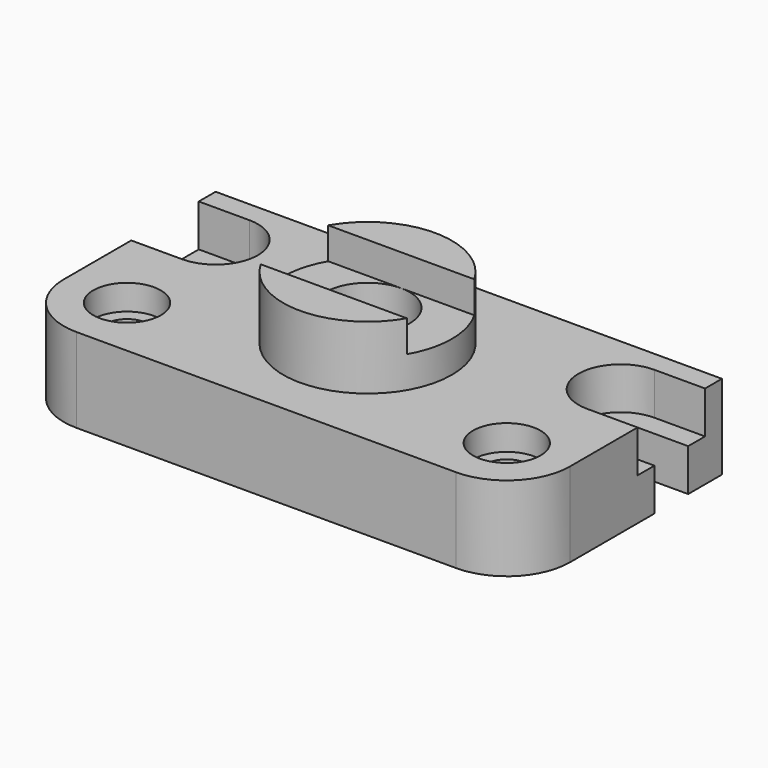
from build123d import *

# Parameters (mm, degrees)
F1_DEPTH        = 20
F2_R            = 20
F3_DEPTH        = 15
F6_DEPTH        = 20.001
F7_DEPTH        = 10
F8_D            = 10
F8_CBORE_D      = 16
F8_CBORE_DEPTH  = 6
F10_D           = 10
F10_CBORE_D     = 20
F10_CBORE_DEPTH = 25
F12_DEPTH       = 7.5


# Not quite as in the source:
# - a feature names something its author has since deleted; it is built from what else it names


with BuildPart() as f1:
    # F0 (on Top) → F1 (new body)
    with BuildSketch(Plane.XY):
        with BuildLine():
            Line((60, 30), (-60, 30))
            Line((-60, 30), (-60, -15))
            ThreePointArc((-60, -15), (-55.6066017178, -25.6066017178), (-45, -30))
            Line((-45, -30), (45, -30))
            ThreePointArc((45, -30), (55.6066017178, -25.6066017178), (60, -15))
            Line((60, -15), (60, 30))
        make_face()
    extrude(amount=F1_DEPTH)

    # F2 (on face) → F3 (join)
    with BuildSketch(Plane.XY.offset(20)):
        Circle(F2_R)
    extrude(amount=F3_DEPTH)

    # F5 (on face) → F6 (cut, through all)
    with BuildSketch(Plane.XY.offset(20)):
        with BuildLine():
            Line((-60, 20), (-60, 10))
            Line((-60, 10), (-48, 10))
            ThreePointArc((-48, 10), (-43, 15), (-48, 20))
            Line((-48, 20), (-60, 20))
        make_face()
        with BuildLine():
            Line((60, 10), (60, 20))
            Line((60, 20), (48, 20))
            ThreePointArc((48, 20), (43, 15), (48, 10))
            Line((48, 10), (60, 10))
        make_face()
    extrude(amount=-F6_DEPTH, mode=Mode.SUBTRACT)

    # F5 (on face) → F7 (cut)
    with BuildSketch(Plane.XY.offset(20)):
        with BuildLine():
            Line((-60, 5), (-48, 5))
            ThreePointArc((-48, 5), (-38, 15), (-48, 25))
            Line((-48, 25), (-60, 25))
            Line((-60, 25), (-60, 20))
            Line((-60, 20), (-48, 20))
            ThreePointArc((-48, 20), (-43, 15), (-48, 10))
            Line((-48, 10), (-60, 10))
            Line((-60, 10), (-60, 5))
        make_face()
        with BuildLine():
            Line((60, 20), (60, 25))
            Line((60, 25), (48, 25))
            ThreePointArc((48, 25), (38, 15), (48, 5))
            Line((48, 5), (60, 5))
            Line((60, 5), (60, 10))
            Line((60, 10), (48, 10))
            ThreePointArc((48, 10), (43, 15), (48, 20))
            Line((48, 20), (60, 20))
        make_face()
    extrude(amount=-F7_DEPTH, mode=Mode.SUBTRACT)

    # F8 (through all)
    with Locations(Plane.XY.offset(20)):
        with Locations((-45, -15), (45, -15)):
            CounterBoreHole(F8_D / 2, F8_CBORE_D / 2, F8_CBORE_DEPTH)

    # F10 (through all)
    with Locations(Plane.XY.offset(35)):
        with Locations((0, 0)):
            CounterBoreHole(F10_D / 2, F10_CBORE_D / 2, F10_CBORE_DEPTH)

    # F11 (on face) → F12 (cut)
    with BuildSketch(Plane.XY.offset(35)):
        with BuildLine():
            Line((-3.73e-08, 10), (-17.3205080757, 10))
            ThreePointArc((-17.3205080757, 10), (-19.3185165265, 5.1763808994), (-20, -5.5e-09))
            ThreePointArc((-20, -5.5e-09), (-19.3185165251, -5.1763809047), (-17.3205080757, -10))
            Line((-17.3205080757, -10), (0, -10))
            ThreePointArc((0, -10), (-10, -1.87e-08), (-3.73e-08, 10))
        make_face()
        with BuildLine():
            Line((17.3205080757, 10), (-3.73e-08, 10))
            ThreePointArc((-3.73e-08, 10), (7.0710677987, 7.0710678251), (10, 0))
            ThreePointArc((10, 0), (7.0710678119, -7.0710678119), (0, -10))
            Line((0, -10), (17.3205080757, -10))
            ThreePointArc((17.3205080757, -10), (19.3185165258, -5.1763809021), (20, 0))
            ThreePointArc((20, 0), (19.3185165258, 5.1763809021), (17.3205080757, 10))
        make_face()
    extrude(amount=-F12_DEPTH, mode=Mode.SUBTRACT)


solid = f1.part
